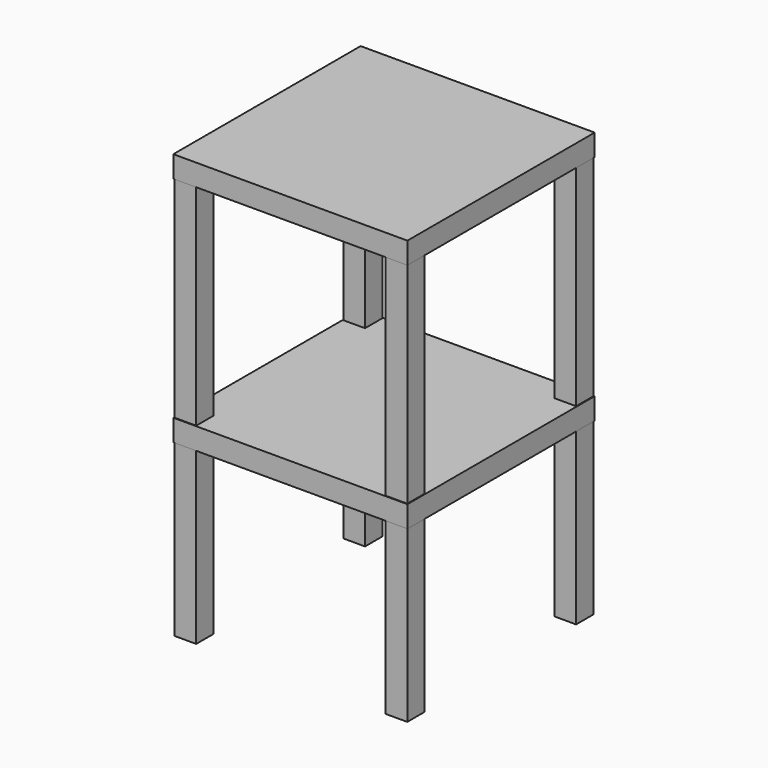
from build123d import *

# Parameters (mm, degrees)
F0_W     = 549.275
F0_H     = 549.275
F1_DEPTH = 50.8
F2_W     = 50.8
F2_H     = 50.8
F3_DEPTH = 400.05
F5_DEPTH = 493.7


with BuildPart() as f1:
    # F0 (on Top) → F1 (new body)
    with BuildSketch(Plane.XY):
        Rectangle(F0_W, F0_H)
    extrude(amount=F1_DEPTH)

    # F2 (on Top) → F3 (join)
    with BuildSketch(Plane.XY):
        with Locations((247.65, -247.65)):
            Rectangle(F2_W, F2_H)
        with Locations((247.65, 247.65)):
            Rectangle(F2_W, F2_H)
        with Locations((-247.65, 247.65)):
            Rectangle(F2_W, F2_H)
        with Locations((-247.65, -247.65)):
            Rectangle(F2_W, F2_H)
    extrude(amount=-F3_DEPTH)


with BuildPart() as f4_1:
    # F4: copy of F1
    add(f1.part.moved(Location((0, 0, -544.5))))


with BuildPart() as f1_1:
    add(f1.part)

    # F2 (on Top) → F5 (join, through all)
    with BuildSketch(Plane.XY):
        with Locations((247.65, -247.65)):
            Rectangle(F2_W, F2_H)
        with Locations((247.65, 247.65)):
            Rectangle(F2_W, F2_H)
        with Locations((-247.65, 247.65)):
            Rectangle(F2_W, F2_H)
        with Locations((-247.65, -247.65)):
            Rectangle(F2_W, F2_H)
    extrude(amount=-F5_DEPTH)


solid = Compound([f4_1.part, f1_1.part])
